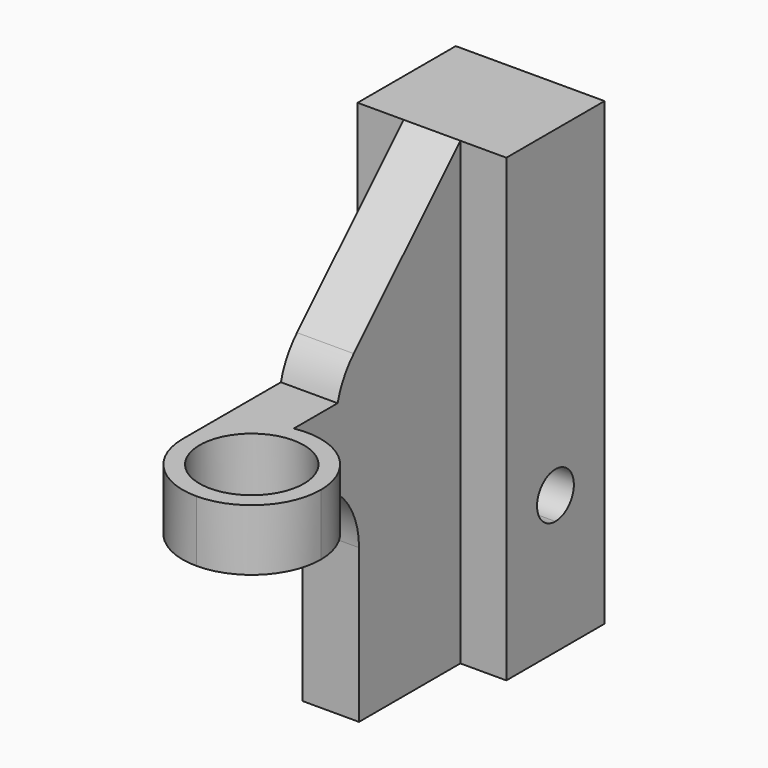
from build123d import *

# Parameters (mm, degrees)
F1_DEPTH     = 19
F3_DEPTH     = 11
F4_R         = 3.4
F5_DEPTH     = 25
F8_DEPTH     = 25
F9_T1_DEPTH  = 55.1336597593
F10_DEPTH    = 15
F11_T1_DEPTH = 3.7
F11_T3_DEPTH = 12.9815131525


# Not quite as in the source:
# - a fillet or chamfer that OpenCascade refuses, or shapes differently, is made with other operations: its cross-section is extruded or revolved along the edge and cut away or added


with BuildPart() as f1:
    # F0 (on Top) → F1 (new body)
    with BuildSketch(Plane.XY):
        with BuildLine():
            ThreePointArc((4, 0), (7.1819805153, 1.3180194847), (8.5, 4.5))
            ThreePointArc((8.5, 4.5), (6.8853076093, 7.95325933), (3.2, 8.9283179651))
            ThreePointArc((3.2, 8.9283179651), (0.54674067, 7.3853076093), (-0.5, 4.5))
            ThreePointArc((-0.5, 4.5), (0.8180194847, 1.3180194847), (4, 0))
        make_face()
        with BuildLine():
            ThreePointArc((-0.5, 4.5), (0.54674067, 7.3853076093), (3.2, 8.9283179651))
            Line((3.2, 8.9283179651), (3.2, 22.5))
            Line((3.2, 22.5), (6.2, 22.5))
            Line((6.2, 22.5), (6.2, 30.5))
            Line((6.2, 30.5), (-3.5, 30.5))
            Line((-3.5, 30.5), (-3.5, 22.5))
            Line((-3.5, 22.5), (-0.5, 22.5))
            Line((-0.5, 22.5), (-0.5, 4.5))
        make_face()
    extrude(amount=F1_DEPTH)

    # F2 (on face) → F3 (join)
    with BuildSketch(Plane.XY.offset(19)):
        Polygon((6.2, 30.5), (-3.5, 30.5), (-3.5, 22.5), (-0.5, 22.5), (-0.5, 12.5), (3.2, 12.5), (3.2, 22.5), (6.2, 22.5), align=None)
    extrude(amount=F3_DEPTH)

    # F4 (on face) → F5 (cut)
    with BuildSketch(Plane(origin=(0, 0, 0), x_dir=(1, 0, 0), z_dir=(0, 0, -1))):
        with Locations((4, -4.5)):
            Circle(F4_R)
    extrude(amount=-F5_DEPTH, mode=Mode.SUBTRACT)

    # F7 (on face) → F8 (cut)
    with BuildSketch(Plane(origin=(-3.5, 0, 0), x_dir=(0, -1, 0), z_dir=(-1, 0, 0))):
        with BuildLine():
            ThreePointArc((-26.5, 7.5), (-25.4393398282, 7.9393398282), (-25, 9))
            ThreePointArc((-25, 9), (-27.5606601718, 10.0606601718), (-26.5, 7.5))
        make_face()
    extrude(amount=-F8_DEPTH, mode=Mode.SUBTRACT)

    # F9: chamfer of 10 on 1 edges, made by hand

    # F9_s2 → F9_t1 (cut)
    with BuildSketch(Plane.YZ.offset(-26.2168298797)):
        Polygon((12.5, 20), (22.5, 30), (12.5, 30), align=None)
    extrude(amount=F9_T1_DEPTH, mode=Mode.SUBTRACT)

    # F6 (on Top) → F10 (cut)
    with BuildSketch(Plane.XY):
        Polygon((-2.952047158, 0), (0, 0), (4.1492179482, 0), (5.4492179482, 0), (9.2530830997, 0), (9.2530830997, 9.0487509014), (9.2530830997, 14.2418248579), (-2.952047158, 14.2418248579), align=None)
    extrude(amount=F10_DEPTH, mode=Mode.SUBTRACT)

    # F11: fillet of radius 5 on 2 edges, made by hand

    # F11_s2 → F11_t1 (join)
    with BuildSketch(Plane.YZ.offset(-0.5)):
        with BuildLine():
            ThreePointArc((14.2418248579, 10), (12.7773587638, 13.5355339059), (9.2418248579, 15))
            Line((9.2418248579, 15), (14.2418248579, 15))
            Line((14.2418248579, 15), (14.2418248579, 10))
        make_face()
    extrude(amount=F11_T1_DEPTH)

    # F11_s4 → F11_t3 (cut)
    with BuildSketch(Plane.YZ.offset(-5.1407565762)):
        with BuildLine():
            ThreePointArc((13.812604178, 21.312604178), (12.9997448715, 20.2451619378), (12.5, 19))
            Line((12.5, 19), (12.5, 20))
            Line((12.5, 20), (13.812604178, 21.312604178))
        make_face()
    extrude(amount=F11_T3_DEPTH, mode=Mode.SUBTRACT)


solid = f1.part
